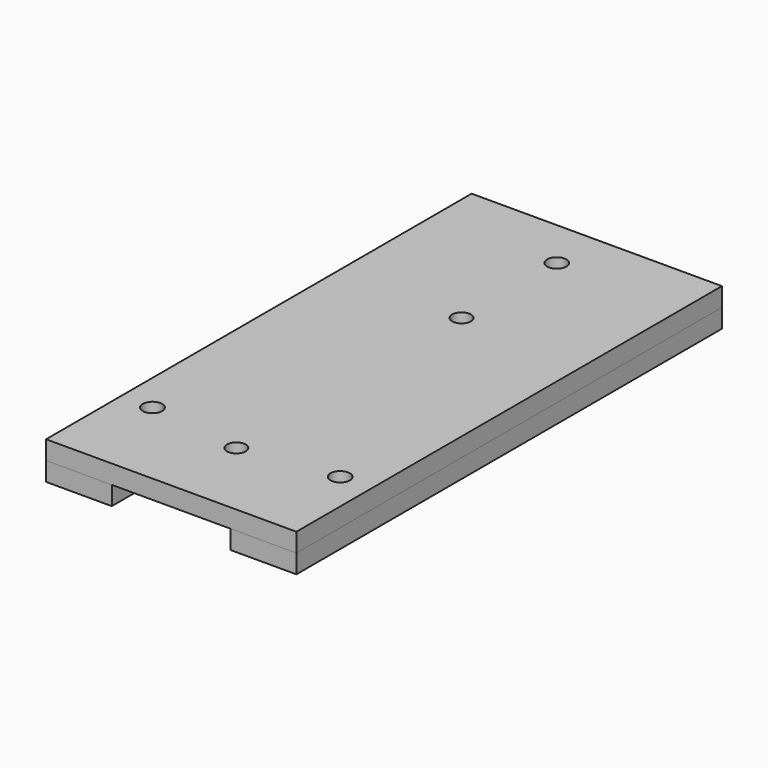
from build123d import *

# Parameters (mm, degrees)
F1_DEPTH = 3
F2_W     = 19
F2_H     = 70
F3_DEPTH = 3
F4_R     = 1.55
F5_DEPTH = 25
F6_R     = 1.5
F7_DEPTH = 25


with BuildPart() as f1:
    # F0 (on Top) → F1 (new body)
    with BuildSketch(Plane.XY):
        Polygon((-9.5, 35), (9.5, 35), (9.5, -35), (20, -35), (20, 50), (-20, 50), (-20, -35), (-9.5, -35), align=None)
    extrude(amount=F1_DEPTH)


with BuildPart() as f3:
    # F2 (on face) → F3 (new body)
    with BuildSketch(Plane.XY.offset(3)):
        Polygon((20, -35), (20, 50), (-20, 50), (-20, -35), (-9.5, -35), (-9.5, 35), (9.5, 35), (9.5, -35), align=None)
        Rectangle(F2_W, F2_H)
    extrude(amount=F3_DEPTH)


with BuildPart() as f5_tool:
    # F4 (on face) → F5 (new body)
    with BuildSketch(Plane.XY.offset(6)):
        with Locations((-15, -20)):
            Circle(F4_R)
        with Locations((15, -20)):
            Circle(F4_R)
        with Locations((0, 42)):
            Circle(F4_R)
    extrude(amount=-F5_DEPTH)


with BuildPart() as f1_1:
    add(f1.part)

    # F5: cut by f5_tool
    add(f5_tool.part, mode=Mode.SUBTRACT)


with BuildPart() as f3_1:
    add(f3.part)

    # F5: cut by f5_tool
    add(f5_tool.part, mode=Mode.SUBTRACT)

    # F6 (on face) → F7 (cut)
    with BuildSketch(Plane(origin=(0, 0, 3), x_dir=(1, 0, 0), z_dir=(0, 0, -1))):
        with Locations((0, -23)):
            Circle(F6_R)
        with Locations((0, 22)):
            Circle(F6_R)
    extrude(amount=-F7_DEPTH, mode=Mode.SUBTRACT)


solid = Compound([f1_1.part, f3_1.part])
